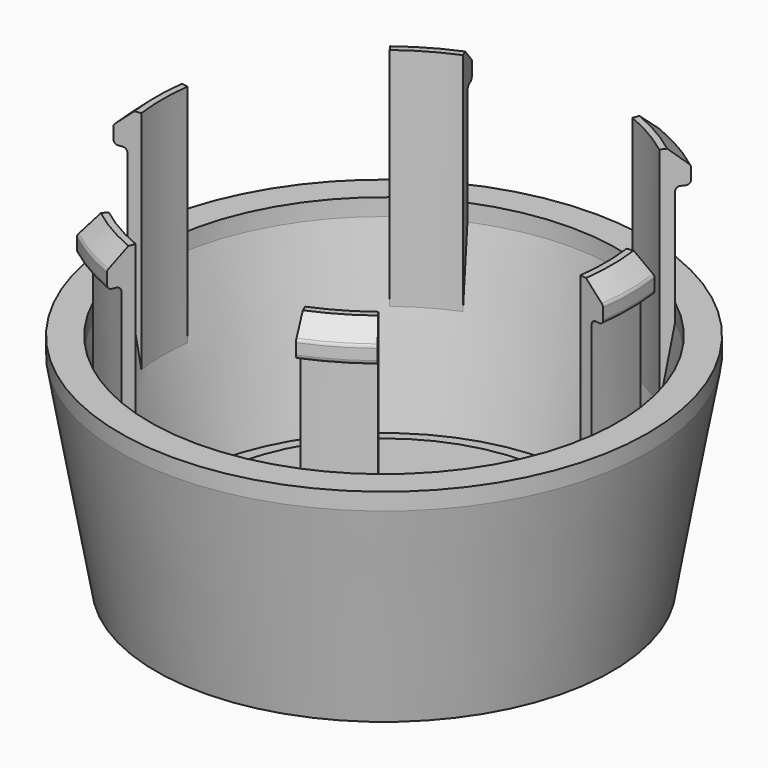
from build123d import *

# Parameters (mm, degrees)
F3_ANGLE_BACK   = 7.5
F3_ANGLE        = 15
F3_COPIES_COUNT = 6
F4_R            = 0.5


# Not quite as in the source:
# - a pattern or mirror of a feature is missing from the dataset's text; its kind, count and spacing are read off the source's solid


with BuildPart() as f1:
    # F0 (on Front) → F1 (revolve)
    with BuildSketch(Plane.XZ):
        Polygon((-24.768152463, 1.5), (0, 1.5), (0, 4.5), (-20.8852968955, 4.5), (-20.8852968955, 3.5), (-23.8852968955, 3.5), (-27.5, 24), (-27.5, 26), (-31, 26), (-31, 24), (-26.768152463, 0), (-24.768152463, 0), align=None)
    revolve(axis=Axis((0, 0, 25), (0, 0, 1)))

    # F2 (on Front) → F3 (revolve)
    with BuildSketch(Plane.XZ, mode=Mode.PRIVATE) as f3_sk:
        Polygon((-27.5, 38), (-27.5, 24), (-26, 15.4930772706), (-26, 42), (-26.75, 42), (-29, 40), (-29, 38), align=None)
    f3 = revolve(f3_sk.sketch.rotate(Axis((0, 0, 25), (0, 0, 1)), -F3_ANGLE_BACK), axis=Axis((0, 0, 25), (0, 0, 1)), revolution_arc=F3_ANGLE)

    # F3_copies: F3 ×6 about axis
    f3_copies_axis = Axis((0, 0, 0), (0, 0, 1))
    for i in range(1, F3_COPIES_COUNT):
        add(f3.rotate(f3_copies_axis, i * 360 / F3_COPIES_COUNT))

    # F4
    f4_edges = [f1.edges().sort_by_distance(p)[0] for p in [
        (-29, 0, 38),
        (-29, 0, 40),
        (-27.5, 0, 38),
        (-13.75, -23.815699, 38),
        (13.75, -23.815699, 38),
        (27.5, 0, 38),
        (13.75, 23.815699, 38),
        (-13.75, 23.815699, 38),
        (-14.5, -25.114737, 38),
        (14.5, -25.114737, 38),
        (29, 0, 38),
        (14.5, 25.114737, 38),
        (-14.5, 25.114737, 38),
        (-14.5, -25.114737, 40),
        (14.5, -25.114737, 40),
        (29, 0, 40),
        (14.5, 25.114737, 40),
        (-14.5, 25.114737, 40),
    ]]
    fillet(f4_edges, radius=F4_R)


solid = f1.part
